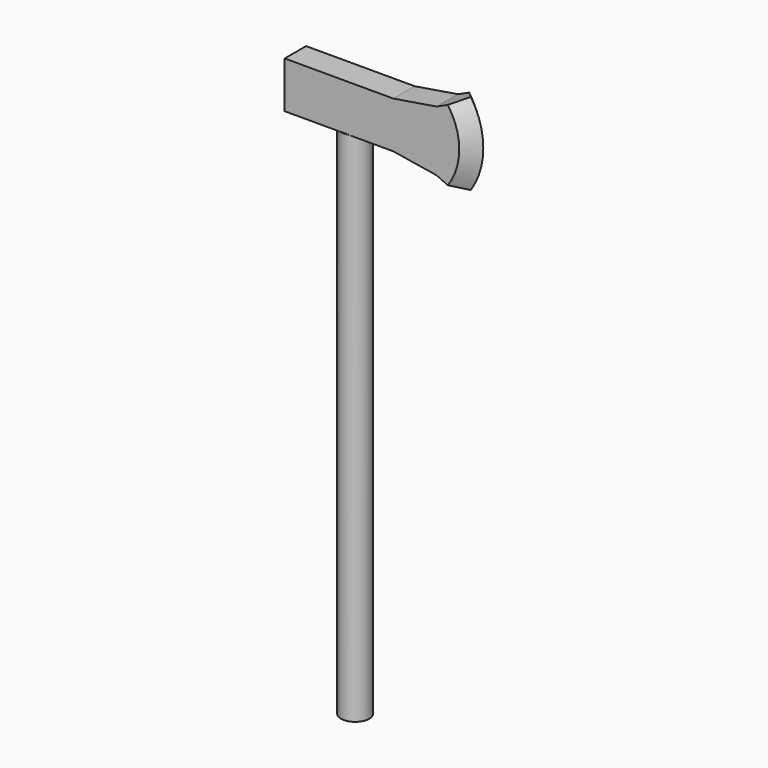
from build123d import *

# Parameters (mm, degrees)
F0_R          = 11.4398919201
F1_DEPTH      = 419.01794
F3_DEPTH      = 10.8458
F3_DEPTH_BACK = 10.84517
F4_T2_ANGLE   = 127.5095974459
F4_T4_ANGLE   = 127.5095974459


# Not quite as in the source:
# - a fillet or chamfer that OpenCascade refuses, or shapes differently, is made with other operations: its cross-section is extruded or revolved along the edge and cut away or added


with BuildPart() as f1:
    # F0 (on Top) → F1 (new body)
    with BuildSketch(Plane.XY):
        Circle(F0_R)
    extrude(amount=F1_DEPTH)

    # F2 (on Front) → F3 (join, two sides)
    with BuildSketch(Plane.XZ) as f3_sk:
        with BuildLine():
            Line((-48.4741501155, 456.7061818215), (-48.4741501155, 418.9741480511))
            Line((-48.4741501155, 418.9741480511), (39.7135697317, 418.9741480511))
            Line((39.7135697317, 418.9741480511), (74.8131631411, 413.270452539))
            Line((74.8131631411, 413.270452539), (95.608628696, 403.7768645791))
            ThreePointArc((95.608628696, 403.7768645791), (105.8473453497, 437.8401649363), (95.608628696, 471.9034652936))
            Line((95.608628696, 471.9034652936), (74.8131631411, 462.4098773337))
            Line((74.8131631411, 462.4098773337), (39.7135697317, 456.7061818215))
            Line((39.7135697317, 456.7061818215), (-48.4741501155, 456.7061818215))
        make_face()
    extrude(amount=F3_DEPTH)
    extrude(f3_sk.sketch, amount=-F3_DEPTH_BACK)

    # F4: chamfer of 12.7 on 2 edges, made by hand

    # F4_s1 → F4_t2 (revolve, cut)
    with BuildSketch(Plane(origin=(209.1067778356, 0, 103.0982793805), x_dir=(0, 1, 0), z_dir=(-0.8969097816, 0, -0.4422135724))):
        Polygon((-10.8458, -324.1347521568), (1.8542, -311.4347521568), (-10.8458, -311.4347521568), align=None)
    revolve(axis=Axis((44.0652005391, -10.8458, 437.8401649363), (0, -1, 0)), revolution_arc=F4_T2_ANGLE, mode=Mode.SUBTRACT)

    # F4_s3 → F4_t4 (revolve, cut)
    with BuildSketch(Plane(origin=(209.1067778356, 0, 103.0982793805), x_dir=(0, 1, 0), z_dir=(-0.8969097816, 0, -0.4422135724))):
        Polygon((10.84517, -324.1347521568), (-1.85483, -311.4347521568), (10.84517, -311.4347521568), align=None)
    revolve(axis=Axis((44.0652005391, 10.84517, 437.8401649363), (0, -1, 0)), revolution_arc=F4_T4_ANGLE, mode=Mode.SUBTRACT)


solid = f1.part
